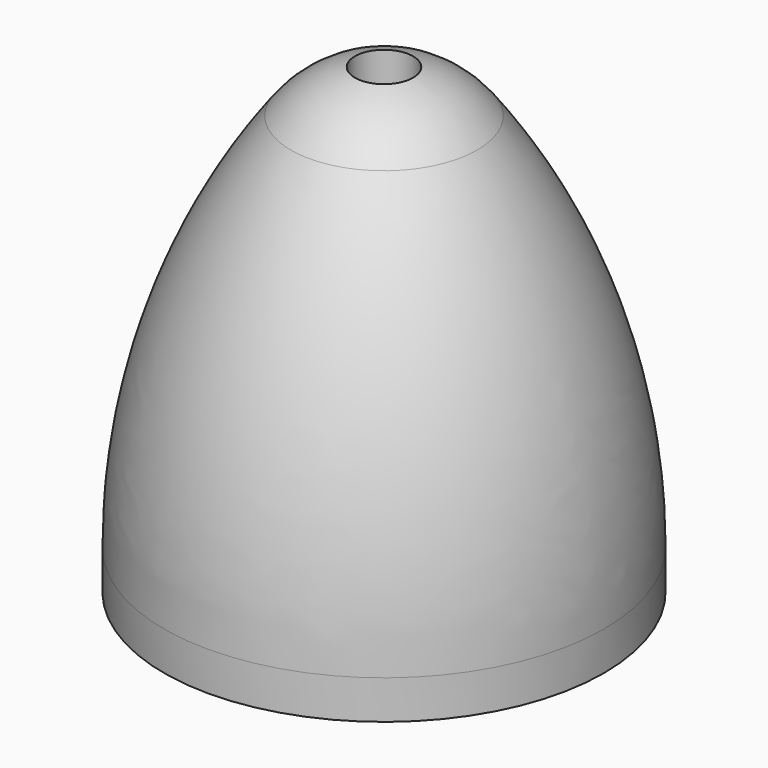
from build123d import *

# Parameters (mm, degrees)
F0_R     = 35.9791
F1_DEPTH = 76.2
F4_R     = 4.7625
F5_DEPTH = 156
F6_R     = 1.7272
F7_DEPTH = 12.7


# Not quite as in the source:
# - an extrude ends at something that could not be found from the text; its depth is read off the source's solid


with BuildPart() as f1:
    # F0 (on Top) → F1 (new body)
    with BuildSketch(Plane.XY):
        Circle(F0_R)
    extrude(amount=F1_DEPTH)

    # F2 (on Front) → F3 (revolve, cut)
    with BuildSketch(Plane.XZ):
        with BuildLine():
            ThreePointArc((0, 76.2), (8.5206969151, 74.1881989682), (15.2417143714, 68.5777138143))
            ThreePointArc((15.2417143714, 68.5777138143), (30.6582935654, 39.1460650432), (35.9791, 6.35))
            Line((35.9791, 6.35), (71.9582, 6.35))
            Line((71.9582, 6.35), (71.9582, 112.1791))
            Line((71.9582, 112.1791), (0, 112.1791))
            Line((0, 112.1791), (0, 76.2))
        make_face()
    revolve(axis=Axis((0, 0, 76.2), (0, 0, 1)), mode=Mode.SUBTRACT)

    # F4 (on face) → F5 (cut, through all)
    with BuildSketch(Plane(origin=(0, 0, 0), x_dir=(1, 0, 0), z_dir=(0, 0, -1))):
        Circle(F4_R)
    extrude(amount=-F5_DEPTH, mode=Mode.SUBTRACT)

    # F6 (on face) → F7 (cut)
    with BuildSketch(Plane(origin=(0, 0, 0), x_dir=(1, 0, 0), z_dir=(0, 0, -1))):
        with Locations((-27.0343686198, -15.6083)):
            Circle(F6_R)
        with Locations((-27.0343686198, 15.6083)):
            Circle(F6_R)
        with Locations((0, 31.2166)):
            Circle(F6_R)
        with Locations((27.0343686198, 15.6083)):
            Circle(F6_R)
        with Locations((27.0343686198, -15.6083)):
            Circle(F6_R)
        with Locations((0, -31.2166)):
            Circle(F6_R)
    extrude(amount=-F7_DEPTH, mode=Mode.SUBTRACT)


solid = f1.part
